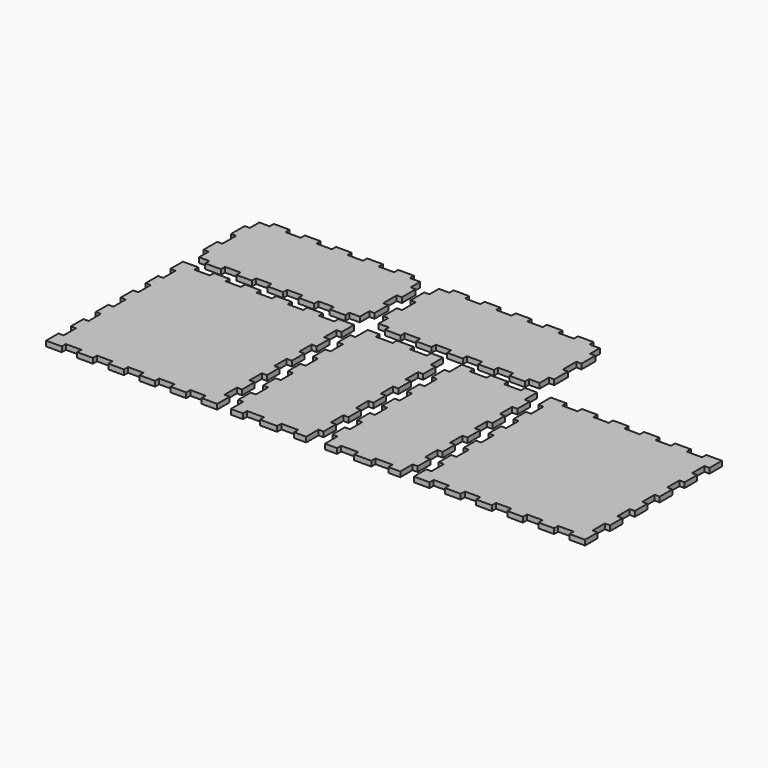
from build123d import *

# Parameters (mm, degrees)
F1_DEPTH = 3


# Not quite as in the source:
# - a feature of the source that left no trace in its solid (it failed there, or was rolled back) is left out


with BuildPart() as f1:
    # F0 (on Top) → F1 (new body)
    with BuildSketch(Plane.XY):
        Polygon((-154.5, -59.398182), (-154.5, -68.409091), (-157.5, -68.409091), (-157.5, -77.5), (-148.329091, -77.5), (-148.329091, -74.5), (-139.318182, -74.5), (-139.318182, -77.5), (-130.147273, -77.5), (-130.147273, -74.5), (-121.136364, -74.5), (-121.136364, -77.5), (-111.965455, -77.5), (-111.965455, -74.5), (-102.954545, -74.5), (-102.954545, -77.5), (-93.783636, -77.5), (-93.783636, -74.5), (-84.772727, -74.5), (-84.772727, -77.5), (-75.601818, -77.5), (-75.601818, -74.5), (-66.590909, -74.5), (-66.590909, -77.5), (-57.5, -77.5), (-57.5, -68.329091), (-60.5, -68.329091), (-60.5, -59.318182), (-57.5, -59.318182), (-57.5, -50.147273), (-60.5, -50.147273), (-60.5, -41.136364), (-57.5, -41.136364), (-57.5, -31.965455), (-60.5, -31.965455), (-60.5, -22.954545), (-57.5, -22.954545), (-57.5, -13.783636), (-60.5, -13.783636), (-60.5, -4.772727), (-57.5, -4.772727), (-57.5, 4.398182), (-60.5, 4.398182), (-60.5, 13.409091), (-57.5, 13.409091), (-57.5, 22.5), (-66.670909, 22.5), (-66.670909, 19.5), (-75.681818, 19.5), (-75.681818, 22.5), (-84.852727, 22.5), (-84.852727, 19.5), (-93.863636, 19.5), (-93.863636, 22.5), (-103.034545, 22.5), (-103.034545, 19.5), (-112.045455, 19.5), (-112.045455, 22.5), (-121.216364, 22.5), (-121.216364, 19.5), (-130.227273, 19.5), (-130.227273, 22.5), (-139.398182, 22.5), (-139.398182, 19.5), (-148.409091, 19.5), (-148.409091, 22.5), (-157.5, 22.5), (-157.5, 13.329091), (-154.5, 13.329091), (-154.5, 4.318182), (-157.5, 4.318182), (-157.5, -4.852727), (-154.5, -4.852727), (-154.5, -13.863636), (-157.5, -13.863636), (-157.5, -23.034545), (-154.5, -23.034545), (-154.5, -32.045455), (-157.5, -32.045455), (-157.5, -41.216364), (-154.5, -41.216364), (-154.5, -50.227273), (-157.5, -50.227273), (-157.5, -59.398182), align=None)
    extrude(amount=F1_DEPTH)


with BuildPart() as f1b:
    # F0 (on Top) → F1, piece 2 (new body)
    with BuildSketch(Plane.XY):
        Polygon((60.5, -59.398182), (60.5, -68.409091), (57.5, -68.409091), (57.5, -77.5), (66.670909, -77.5), (66.670909, -74.5), (75.681818, -74.5), (75.681818, -77.5), (84.852727, -77.5), (84.852727, -74.5), (93.863636, -74.5), (93.863636, -77.5), (103.034545, -77.5), (103.034545, -74.5), (112.045455, -74.5), (112.045455, -77.5), (121.216364, -77.5), (121.216364, -74.5), (130.227273, -74.5), (130.227273, -77.5), (139.398182, -77.5), (139.398182, -74.5), (148.409091, -74.5), (148.409091, -77.5), (157.5, -77.5), (157.5, -68.329091), (154.5, -68.329091), (154.5, -59.318182), (157.5, -59.318182), (157.5, -50.147273), (154.5, -50.147273), (154.5, -41.136364), (157.5, -41.136364), (157.5, -31.965455), (154.5, -31.965455), (154.5, -22.954545), (157.5, -22.954545), (157.5, -13.783636), (154.5, -13.783636), (154.5, -4.772727), (157.5, -4.772727), (157.5, 4.398182), (154.5, 4.398182), (154.5, 13.409091), (157.5, 13.409091), (157.5, 22.5), (148.329091, 22.5), (148.329091, 19.5), (139.318182, 19.5), (139.318182, 22.5), (130.147273, 22.5), (130.147273, 19.5), (121.136364, 19.5), (121.136364, 22.5), (111.965455, 22.5), (111.965455, 19.5), (102.954545, 19.5), (102.954545, 22.5), (93.783636, 22.5), (93.783636, 19.5), (84.772727, 19.5), (84.772727, 22.5), (75.601818, 22.5), (75.601818, 19.5), (66.590909, 19.5), (66.590909, 22.5), (57.5, 22.5), (57.5, 13.329091), (60.5, 13.329091), (60.5, 4.318182), (57.5, 4.318182), (57.5, -4.852727), (60.5, -4.852727), (60.5, -13.863636), (57.5, -13.863636), (57.5, -23.034545), (60.5, -23.034545), (60.5, -32.045455), (57.5, -32.045455), (57.5, -41.216364), (60.5, -41.216364), (60.5, -50.227273), (57.5, -50.227273), (57.5, -59.398182), align=None)
    extrude(amount=F1_DEPTH)


with BuildPart() as f1c:
    # F0 (on Top) → F1, piece 3 (new body)
    with BuildSketch(Plane.XY):
        Polygon((-154.5, 47.58), (-157.5, 47.58), (-157.5, 37.5), (-154.5, 37.5), (-154.5, 30.5), (-148.489091, 30.5), (-148.489091, 27.5), (-139.318182, 27.5), (-139.318182, 30.5), (-130.307273, 30.5), (-130.307273, 27.5), (-121.136364, 27.5), (-121.136364, 30.5), (-112.125455, 30.5), (-112.125455, 27.5), (-102.954545, 27.5), (-102.954545, 30.5), (-93.943636, 30.5), (-93.943636, 27.5), (-84.772727, 27.5), (-84.772727, 30.5), (-75.761818, 30.5), (-75.761818, 27.5), (-66.590909, 27.5), (-66.590909, 30.5), (-60.5, 30.5), (-60.5, 37.42), (-57.5, 37.42), (-57.5, 47.5), (-60.5, 47.5), (-60.5, 57.42), (-57.5, 57.42), (-57.5, 67.5), (-60.5, 67.5), (-60.5, 74.5), (-66.510909, 74.5), (-66.510909, 77.5), (-75.681818, 77.5), (-75.681818, 74.5), (-84.692727, 74.5), (-84.692727, 77.5), (-93.863636, 77.5), (-93.863636, 74.5), (-102.874545, 74.5), (-102.874545, 77.5), (-112.045455, 77.5), (-112.045455, 74.5), (-121.056364, 74.5), (-121.056364, 77.5), (-130.227273, 77.5), (-130.227273, 74.5), (-139.238182, 74.5), (-139.238182, 77.5), (-148.409091, 77.5), (-148.409091, 74.5), (-154.5, 74.5), (-154.5, 67.58), (-157.5, 67.58), (-157.5, 57.5), (-154.5, 57.5), align=None)
    extrude(amount=F1_DEPTH)


with BuildPart() as f1d:
    # F0 (on Top) → F1, piece 4 (new body)
    with BuildSketch(Plane.XY):
        Polygon((-49.5, -68.409091), (-49.5, -77.5), (-42.42, -77.5), (-42.42, -74.5), (-32.5, -74.5), (-32.5, -77.5), (-22.42, -77.5), (-22.42, -74.5), (-12.5, -74.5), (-12.5, -77.5), (-5.5, -77.5), (-5.5, -68.489091), (-2.5, -68.489091), (-2.5, -59.318182), (-5.5, -59.318182), (-5.5, -50.307273), (-2.5, -50.307273), (-2.5, -41.136364), (-5.5, -41.136364), (-5.5, -32.125455), (-2.5, -32.125455), (-2.5, -22.954545), (-5.5, -22.954545), (-5.5, -13.943636), (-2.5, -13.943636), (-2.5, -4.772727), (-5.5, -4.772727), (-5.5, 4.238182), (-2.5, 4.238182), (-2.5, 13.409091), (-5.5, 13.409091), (-5.5, 22.5), (-12.58, 22.5), (-12.58, 19.5), (-22.5, 19.5), (-22.5, 22.5), (-32.58, 22.5), (-32.58, 19.5), (-42.5, 19.5), (-42.5, 22.5), (-49.5, 22.5), (-49.5, 13.489091), (-52.5, 13.489091), (-52.5, 4.318182), (-49.5, 4.318182), (-49.5, -4.692727), (-52.5, -4.692727), (-52.5, -13.863636), (-49.5, -13.863636), (-49.5, -22.874545), (-52.5, -22.874545), (-52.5, -32.045455), (-49.5, -32.045455), (-49.5, -41.056364), (-52.5, -41.056364), (-52.5, -50.227273), (-49.5, -50.227273), (-49.5, -59.238182), (-52.5, -59.238182), (-52.5, -68.409091), align=None)
    extrude(amount=F1_DEPTH)


with BuildPart() as f1e:
    # F0 (on Top) → F1, piece 5 (new body)
    with BuildSketch(Plane.XY):
        Polygon((5.5, -68.409091), (5.5, -77.5), (12.58, -77.5), (12.58, -74.5), (22.5, -74.5), (22.5, -77.5), (32.58, -77.5), (32.58, -74.5), (42.5, -74.5), (42.5, -77.5), (49.5, -77.5), (49.5, -68.489091), (52.5, -68.489091), (52.5, -59.318182), (49.5, -59.318182), (49.5, -50.307273), (52.5, -50.307273), (52.5, -41.136364), (49.5, -41.136364), (49.5, -32.125455), (52.5, -32.125455), (52.5, -22.954545), (49.5, -22.954545), (49.5, -13.943636), (52.5, -13.943636), (52.5, -4.772727), (49.5, -4.772727), (49.5, 4.238182), (52.5, 4.238182), (52.5, 13.409091), (49.5, 13.409091), (49.5, 22.5), (42.42, 22.5), (42.42, 19.5), (32.5, 19.5), (32.5, 22.5), (22.42, 22.5), (22.42, 19.5), (12.5, 19.5), (12.5, 22.5), (5.5, 22.5), (5.5, 13.489091), (2.5, 13.489091), (2.5, 4.318182), (5.5, 4.318182), (5.5, -4.692727), (2.5, -4.692727), (2.5, -13.863636), (5.5, -13.863636), (5.5, -22.874545), (2.5, -22.874545), (2.5, -32.045455), (5.5, -32.045455), (5.5, -41.056364), (2.5, -41.056364), (2.5, -50.227273), (5.5, -50.227273), (5.5, -59.238182), (2.5, -59.238182), (2.5, -68.409091), align=None)
    extrude(amount=F1_DEPTH)


with BuildPart() as f1f:
    # F0 (on Top) → F1, piece 6 (new body)
    with BuildSketch(Plane.XY):
        Polygon((-49.5, 47.58), (-52.5, 47.58), (-52.5, 37.5), (-49.5, 37.5), (-49.5, 30.5), (-43.489091, 30.5), (-43.489091, 27.5), (-34.318182, 27.5), (-34.318182, 30.5), (-25.307273, 30.5), (-25.307273, 27.5), (-16.136364, 27.5), (-16.136364, 30.5), (-7.125455, 30.5), (-7.125455, 27.5), (2.045455, 27.5), (2.045455, 30.5), (11.056364, 30.5), (11.056364, 27.5), (20.227273, 27.5), (20.227273, 30.5), (29.238182, 30.5), (29.238182, 27.5), (38.409091, 27.5), (38.409091, 30.5), (44.5, 30.5), (44.5, 37.42), (47.5, 37.42), (47.5, 47.5), (44.5, 47.5), (44.5, 57.42), (47.5, 57.42), (47.5, 67.5), (44.5, 67.5), (44.5, 74.5), (38.489091, 74.5), (38.489091, 77.5), (29.318182, 77.5), (29.318182, 74.5), (20.307273, 74.5), (20.307273, 77.5), (11.136364, 77.5), (11.136364, 74.5), (2.125455, 74.5), (2.125455, 77.5), (-7.045455, 77.5), (-7.045455, 74.5), (-16.056364, 74.5), (-16.056364, 77.5), (-25.227273, 77.5), (-25.227273, 74.5), (-34.238182, 74.5), (-34.238182, 77.5), (-43.409091, 77.5), (-43.409091, 74.5), (-49.5, 74.5), (-49.5, 67.58), (-52.5, 67.58), (-52.5, 57.5), (-49.5, 57.5), align=None)
    extrude(amount=F1_DEPTH)


solid = Compound([f1.part, f1b.part, f1c.part, f1d.part, f1e.part, f1f.part])
